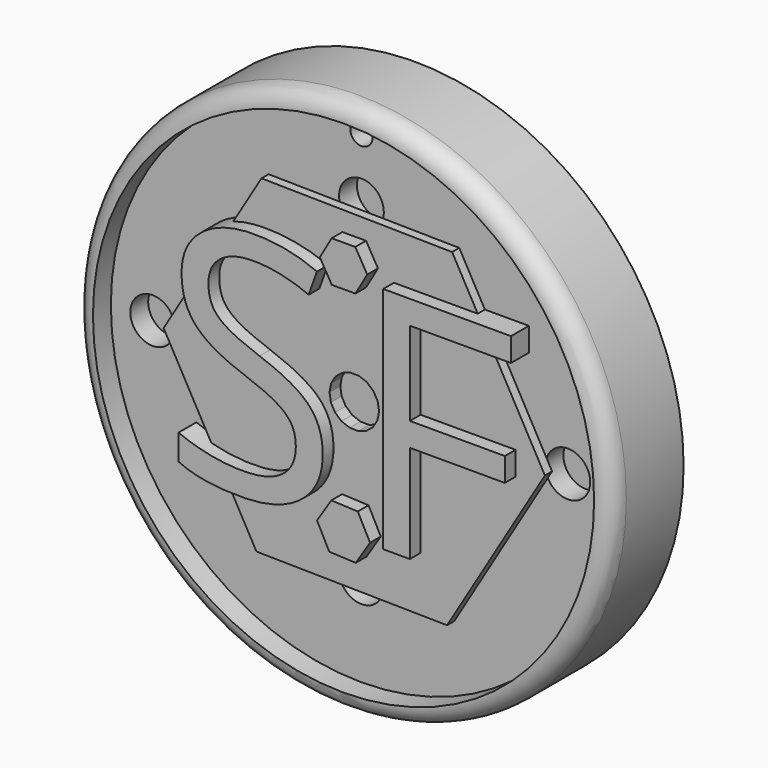
from build123d import *

# Parameters (mm, degrees)
F0_R         = 76.2
F1_DEPTH     = 25.4
F2_R         = 5.08
F3_DEPTH     = 6.35
F4_TEXT_SIZE = 91.0860667419
F5_DEPTH     = 6.35
F6_TEXT_SIZE = 91.0860641549
F7_DEPTH     = 6.35
F8_R         = 3.175
F9_DEPTH     = 50.8
F10_R        = 6.35
F11_DEPTH    = 6.35
F12_R        = 6.35
F13_DEPTH    = 6.35
F14_R        = 6.35
F15_DEPTH    = 6.35
F16_R        = 6.3542300714
F17_DEPTH    = 6.35
F20_DEPTH    = 2.54
F22_DEPTH    = 3.81
F24_DEPTH    = 3.81
F26_DEPTH    = 3.81


# Not quite as in the source:
# - Text() gives the source's letters only with a copy of the font that has no kerning and outlines rounded to 1/6400 em; it was checked with that copy


with BuildPart() as f1:
    # F0 (on Front) → F1 (new body)
    with BuildSketch(Plane.XZ):
        Circle(F0_R)
    extrude(amount=F1_DEPTH)

    # F2
    f2_edges = [f1.edges().sort_by_distance(p)[0] for p in [
        (-76.2, -25.4, 0),
    ]]
    fillet(f2_edges, radius=F2_R)

    # F3 (cut): a face of the model
    f3_faces = [f1.faces().sort_by_distance(p)[0] for p in [
        (0, -25.4, 0),
    ]]
    extrude(f3_faces, amount=-F3_DEPTH, mode=Mode.SUBTRACT)

    # F4 (on face) → F5 (join)
    with BuildSketch(Plane.XZ.offset(19.05)):
        with Locations((-51.5347886988, -30.7506565005)):
            Text('S', F4_TEXT_SIZE, font='Open Sans', text_align=(TextAlign.LEFT, TextAlign.BOTTOM))
    extrude(amount=F5_DEPTH)

    # F6 (on face) → F7 (join)
    with BuildSketch(Plane.XZ.offset(19.05)):
        with Locations((2.3318058811, -31.6250808537)):
            Text('F', F6_TEXT_SIZE, font='Open Sans', text_align=(TextAlign.LEFT, TextAlign.BOTTOM))
    extrude(amount=F7_DEPTH)

    # F8 (on face) → F9 (cut)
    with BuildSketch(Plane.XZ.offset(19.05)):
        with Locations((0, 66.04)):
            Circle(F8_R)
    extrude(amount=-F9_DEPTH, mode=Mode.SUBTRACT)

    # F10 (on face) → F11 (cut)
    with BuildSketch(Plane.XZ.offset(19.05)):
        with Locations((0, 48.384968681)):
            Circle(F10_R)
    extrude(amount=-F11_DEPTH, mode=Mode.SUBTRACT)

    # F12 (on face) → F13 (cut)
    with BuildSketch(Plane.XZ.offset(19.05)):
        with Locations((0, -45.2370159683)):
            Circle(F12_R)
    extrude(amount=-F13_DEPTH, mode=Mode.SUBTRACT)

    # F14 (on face) → F15 (cut)
    with BuildSketch(Plane.XZ.offset(19.05)):
        with Locations((-59.2498590265, 0)):
            Circle(F14_R)
    extrude(amount=-F15_DEPTH, mode=Mode.SUBTRACT)

    # F16 (on face) → F17 (cut)
    with BuildSketch(Plane.XZ.offset(19.05)):
        with Locations((58.5865601897, 0)):
            Circle(F16_R)
    extrude(amount=-F17_DEPTH, mode=Mode.SUBTRACT)

    # F19 (on face) → F20 (join)
    with BuildSketch(Plane.XZ.offset(19.05)):
        Polygon((26.3402288501, -47.2698327996), (54.1069904621, -0.8236090742), (27.7667616121, 46.4462237255), (-26.3402288501, 47.2698327996), (-54.1069904621, 0.8236090742), (-27.7667616121, -46.4462237255), align=None)
    extrude(amount=F20_DEPTH)

    # F21 (on face) → F22 (cut)
    with BuildSketch(Plane.XZ.offset(21.59)):
        Polygon((5.3150014525, -4.5994673933), (6.5675781415, -2.5042480104), (7.0280079794, -0.1069793588), (6.6407563327, 2.3031925824), (5.4525314651, 4.4355655066), (3.6066508321, 6.0329437688), (1.3257548802, 6.9026599757), (-1.1150466763, 6.9398135171), (-3.4213571473, 6.1399231276), (-5.3150014525, 4.5994673933), (-6.5675781415, 2.5042480104), (-7.0280079794, 0.1069793588), (-6.6407563327, -2.3031925824), (-5.4525314651, -4.4355655066), (-3.6066508321, -6.0329437688), (-1.3257548802, -6.9026599757), (1.1150466763, -6.9398135171), (3.4213571473, -6.1399231276), align=None)
    extrude(amount=-F22_DEPTH, mode=Mode.SUBTRACT)

    # F23 (on face) → F24 (join)
    with BuildSketch(Plane.XZ.offset(21.59)):
        Polygon((-4.055395302, -37.2280363057), (3.466013819, -37.5683158636), (7.521409121, -31.2247242715), (4.055395302, -24.5408531215), (-3.466013819, -24.2005735636), (-7.521409121, -30.5441651557), align=None)
    extrude(amount=F24_DEPTH)

    # F25 (on face) → F26 (join)
    with BuildSketch(Plane.XZ.offset(21.59)):
        Polygon((3.3762851661, 29.6899973667), (6.7195147276, 35.518810153), (3.3432295615, 41.3285382771), (-3.3762851661, 41.3094536149), (-6.7195147276, 35.4806408286), (-3.3432295615, 29.6709127045), align=None)
    extrude(amount=F26_DEPTH)


solid = f1.part
